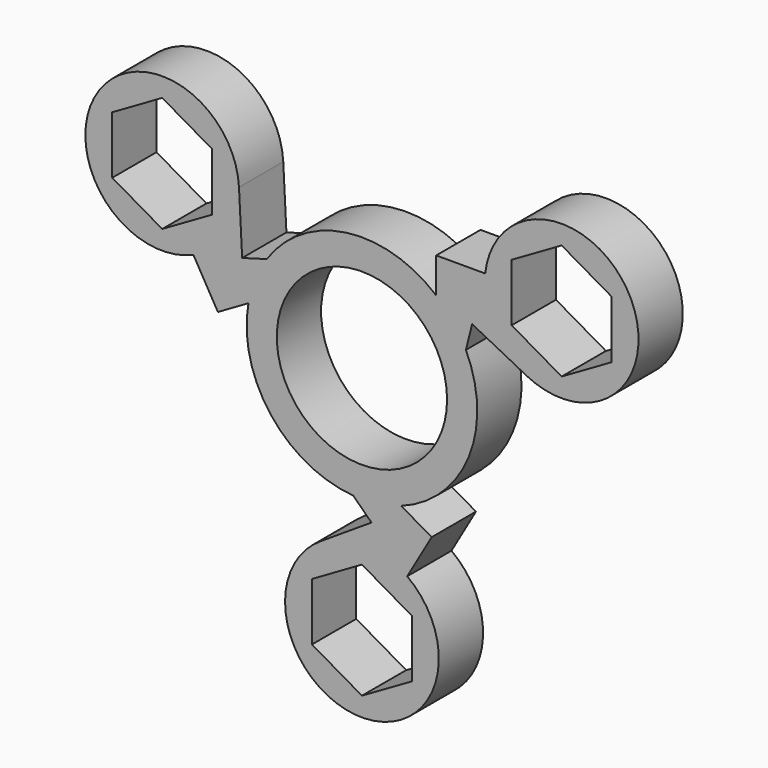
from build123d import *

# Parameters (mm, degrees)
F0_R     = 11.075
F1_DEPTH = 3.6


# Not quite as in the source:
# - a feature of the source that left no trace in its solid (it failed there, or was rolled back) is left out


with BuildPart() as f1:
    # F0 (on Front) → F1 (new body, symmetric)
    with BuildSketch(Plane.XZ):
        with BuildLine():
            Line((-18.7389361234, 0.3405199539), (-14.7669712633, 2.6337349351))
            ThreePointArc((-14.7669712633, 2.6337349351), (-11.8584662517, -9.1856833256), (-1.1413957778, -14.9565108123))
            Line((-1.1413957778, -14.9565108123), (1.2456877462, -17.2733709451))
            Line((1.2456877462, -17.2733709451), (-5.4411288371, -21.6098797995))
            ThreePointArc((-5.4411288371, -21.6098797995), (-0.2713631395, -39.9963174243), (5.8883015494, -21.9174320378))
            Line((5.8883015494, -21.9174320378), (9.0745691311, -16.3986546997))
            Line((9.0745691311, -16.3986546997), (5.102604271, -14.1054397185))
            ThreePointArc((5.102604271, -14.1054397185), (13.8842682369, -5.6768913611), (13.5234162043, 6.4897776668))
            Line((13.5234162043, 6.4897776668), (14.3363341744, 9.7154827059))
            Line((14.3363341744, 9.7154827059), (21.4352692976, 6.0927841016))
            ThreePointArc((21.4352692976, 6.0927841016), (34.773508517, 19.7631513397), (16.0369021558, 16.0581347458))
            Line((16.0369021558, 16.0581347458), (9.6643669923, 16.0581347458))
            Line((9.6643669923, 16.0581347458), (9.6643669923, 11.4717047835))
            ThreePointArc((9.6643669923, 11.4717047835), (-2.0258019852, 14.8625746867), (-12.3820204265, 8.4667331455))
            Line((-12.3820204265, 8.4667331455), (-15.5820219205, 7.5578882392))
            Line((-15.5820219205, 7.5578882392), (-15.9941404606, 15.5170956979))
            ThreePointArc((-15.9941404606, 15.5170956979), (-34.5021453775, 20.2331660846), (-21.9252037051, 5.859297292))
            Line((-21.9252037051, 5.859297292), (-18.7389361234, 0.3405199539))
        make_face()
        Polygon((0, -22.4944465005), (6.5, -26.2472232503), (6.5, -33.7527767497), (0, -37.5055534995), (-6.5, -33.7527767497), (-6.5, -26.2472232503), align=None, mode=Mode.SUBTRACT)
        Circle(F0_R, mode=Mode.SUBTRACT)
        Polygon((-32.4807621135, 11.2472232503), (-32.4807621135, 18.7527767497), (-25.9807621135, 22.5055534995), (-19.4807621135, 18.7527767497), (-19.4807621135, 11.2472232503), (-25.9807621135, 7.4944465005), align=None, mode=Mode.SUBTRACT)
        Polygon((25.9807621135, 22.5055534995), (32.4807621135, 18.7527767497), (32.4807621135, 11.2472232503), (25.9807621135, 7.4944465005), (19.4807621135, 11.2472232503), (19.4807621135, 18.7527767497), align=None, mode=Mode.SUBTRACT)
    extrude(amount=F1_DEPTH, both=True)


solid = f1.part
